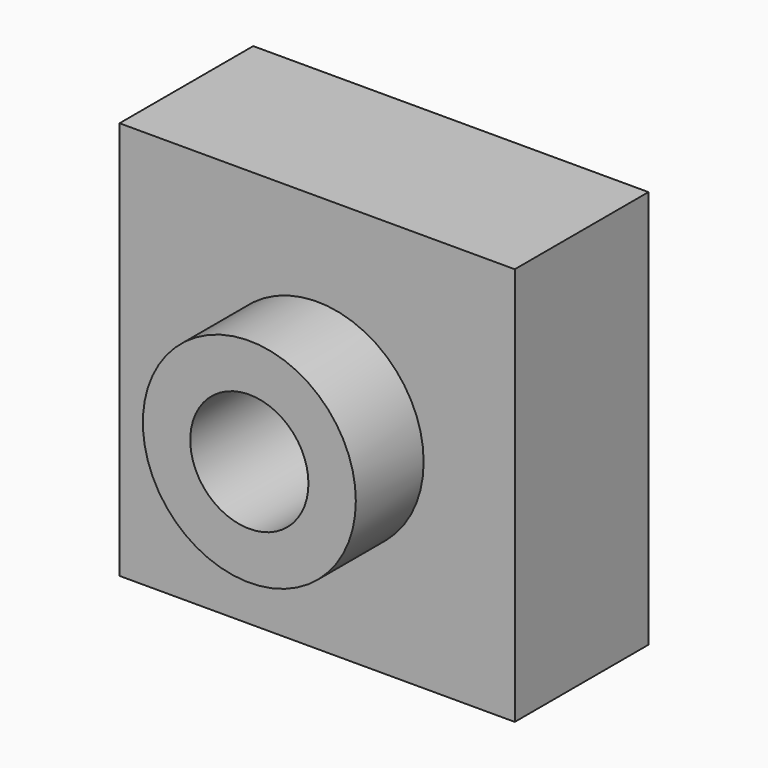
from build123d import *

# Parameters (mm, degrees)
F0_W     = 81.7074924707
F0_H     = 82.3852196336
F0_R     = 22.0154906443
F1_DEPTH = 34.544
F0_R_2   = 12.2186254277
F2_DEPTH = 52.07
F3_DEPTH = 147


# Not quite as in the source:
# - an extrude ends at something that could not be found from the text; its depth is read off the source's solid


with BuildPart() as f1:
    # F0 (on Front) → F1 (new body)
    with BuildSketch(Plane.XZ):
        Rectangle(F0_W, F0_H)
        Circle(F0_R, mode=Mode.SUBTRACT)
    extrude(amount=F1_DEPTH)

    # F0 (on Front) → F2 (join)
    with BuildSketch(Plane.XZ):
        Circle(F0_R)
        Circle(F0_R_2, mode=Mode.SUBTRACT)
    extrude(amount=F2_DEPTH)

    # F0 (on Front) → F3 (cut, through all)
    with BuildSketch(Plane.XZ):
        Circle(F0_R_2)
    extrude(amount=-F3_DEPTH, mode=Mode.SUBTRACT)


solid = f1.part
